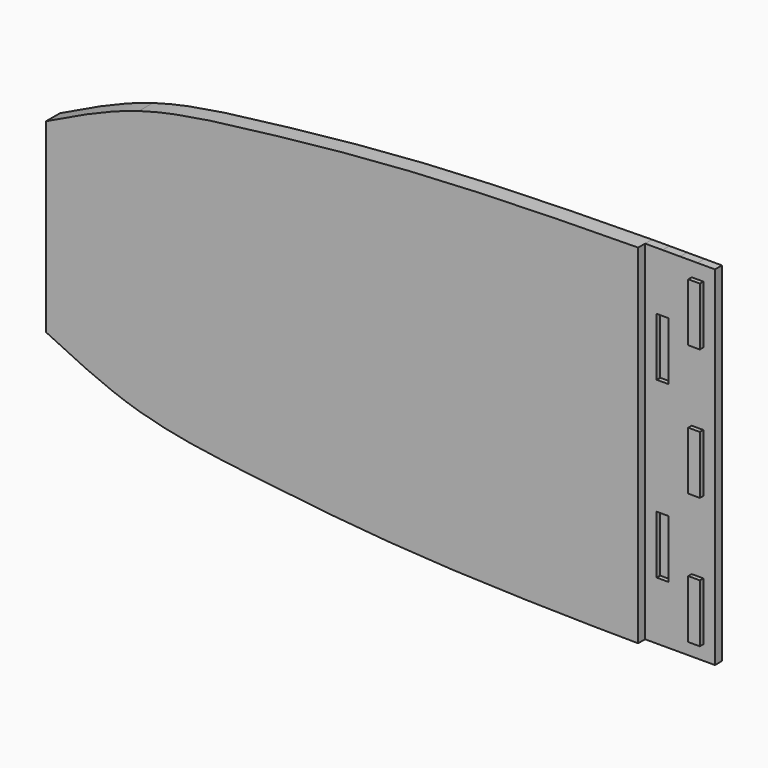
from build123d import *

# Parameters (mm, degrees)
F1_DEPTH = 19.05
F2_DEPTH = 9.525
F0_W     = 6.35
F0_H     = 63.5
F3_DEPTH = 4.7625
F0_H_2   = 31.75
F4_DEPTH = 14.2875


with BuildPart() as f1:
    # F0 (on Front) → F1 (new body)
    with BuildSketch(Plane.XZ):
        with BuildLine():
            Line((-722.3111987114, 1.2279e-06), (-620.7111987114, 1.2279e-06))
            Line((-620.7111987114, 1.2279e-06), (-620.7111987114, 144.4625012279))
            add(Edge.make_bspline(
                [(-722.3111987114, 101.6000012279), (-689.4180363188, 117.6879881372), (-656.5248739262, 133.7759750465), (-620.7111987114, 144.4625012279)],
                knots=[0, 0, 0, 0, 0.1537268507, 0.1537268507, 0.1537268507, 0.1537268507], degree=3))
            Line((-722.3111987114, 101.6000012279), (-722.3111987114, 1.2279e-06))
        make_face()
        with BuildLine():
            Line((-620.7111987114, 1.2279e-06), (-493.7111987114, 1.2279e-06))
            Line((-493.7111987114, 1.2279e-06), (-493.7111987114, 166.6875012279))
            add(Edge.make_bspline(
                [(-620.7111987114, 144.4625012279), (-581.9859047534, 156.0178321253), (-539.8459247327, 161.2577335799), (-493.7111987114, 166.6875012279)],
                knots=[0.1537268507, 0.1537268507, 0.1537268507, 0.1537268507, 0.3199515525, 0.3199515525, 0.3199515525, 0.3199515525], degree=3))
            Line((-620.7111987114, 144.4625012279), (-620.7111987114, 1.2279e-06))
        make_face()
        with BuildLine():
            Line((-620.7111987114, -144.4624987721), (-620.7111987114, 1.2279e-06))
            Line((-620.7111987114, 1.2279e-06), (-722.3111987114, 1.2279e-06))
            Line((-722.3111987114, 1.2279e-06), (-722.3111987114, -101.5999987721))
            add(Edge.make_bspline(
                [(-722.3111987114, -101.5999987721), (-689.4182841733, -117.6941564691), (-656.5253696352, -133.7883141661), (-620.7111987114, -144.4624987721)],
                knots=[0, 0, 0, 0, 0.1537255771, 0.1537255771, 0.1537255771, 0.1537255771], degree=3))
        make_face()
        with BuildLine():
            Line((-493.7111987114, -166.6874987721), (-493.7111987114, 1.2279e-06))
            Line((-493.7111987114, 1.2279e-06), (-620.7111987114, 1.2279e-06))
            Line((-620.7111987114, 1.2279e-06), (-620.7111987114, -144.4624987721))
            add(Edge.make_bspline(
                [(-620.7111987114, -144.4624987721), (-581.9853687438, -156.0044847356), (-539.8439833334, -161.2093964589), (-493.7111987114, -166.6874987721)],
                knots=[0.1537255771, 0.1537255771, 0.1537255771, 0.1537255771, 0.3199489018, 0.3199489018, 0.3199489018, 0.3199489018], degree=3))
        make_face()
        with BuildLine():
            Line((-290.9272084468, -185.0685181572), (-290.9272084468, -0.1247681572))
            Line((-290.9272084468, -0.1247681572), (-290.9272084468, 1.2279e-06))
            Line((-290.9272084468, 1.2279e-06), (-493.7111987114, 1.2279e-06))
            Line((-493.7111987114, 1.2279e-06), (-493.7111987114, -166.6874987721))
            add(Edge.make_bspline(
                [(-493.7111987114, -166.6874987721), (-435.736581071, -173.5717761816), (-371.4584655156, -180.8874953545), (-290.9272084468, -185.0685181572)],
                knots=[0.3199489018, 0.3199489018, 0.3199489018, 0.3199489018, 0.5288401224, 0.5288401224, 0.5288401224, 0.5288401224], degree=3))
        make_face()
        with BuildLine():
            Line((-493.7111987114, 1.2279e-06), (-290.9272084468, 1.2279e-06))
            Line((-290.9272084468, 1.2279e-06), (-290.9272084468, 184.8189818428))
            add(Edge.make_bspline(
                [(-493.7111987114, 166.6875012279), (-435.7373269286, 173.5106620133), (-371.4553650094, 180.633639874), (-290.9272084468, 184.8189818428)],
                knots=[0.3199515525, 0.3199515525, 0.3199515525, 0.3199515525, 0.528833026, 0.528833026, 0.528833026, 0.528833026], degree=3))
            Line((-493.7111987114, 166.6875012279), (-493.7111987114, 1.2279e-06))
        make_face()
        with BuildLine():
            Line((-290.9272084468, 184.8189818428), (-290.9272084468, 1.2279e-06))
            Line((-290.9272084468, 1.2279e-06), (-74.8163211554, 1.2279e-06))
            Line((-74.8163211554, 1.2279e-06), (-74.8163211554, 190.5000012279))
            add(Edge.make_bspline(
                [(-290.9272084468, 184.8189818428), (-207.9460116468, 189.1318172586), (-107.7137651743, 190.3253189595), (-74.8163211554, 190.5000012279)],
                knots=[0.528833026, 0.528833026, 0.528833026, 0.528833026, 0.744077425, 0.744077425, 0.744077425, 0.744077425], degree=3))
        make_face()
        with BuildLine():
            Line((-290.9272084468, 1.2279e-06), (-290.9272084468, -0.1247681572))
            Line((-290.9272084468, -0.1247681572), (-290.9272084468, -185.0685181572))
            add(Edge.make_bspline(
                [(-290.9272084468, -185.0685181572), (-207.9486072246, -189.376602204), (-107.7139882364, -190.35656804), (-74.8163211554, -190.4999987721)],
                knots=[0.5288401224, 0.5288401224, 0.5288401224, 0.5288401224, 0.7440795453, 0.7440795453, 0.7440795453, 0.7440795453], degree=3))
            Line((-74.8163211554, -190.4999987721), (-74.8163211554, 1.2279e-06))
            Line((-74.8163211554, 1.2279e-06), (-290.9272084468, 1.2279e-06))
        make_face()
    extrude(amount=F1_DEPTH)

    # F0 (on Front) → F2 (join)
    with BuildSketch(Plane.XZ):
        Polygon((-74.8163211554, 190.5000012279), (-74.8163211554, 1.2279e-06), (-55.7663211554, 1.2279e-06), (-55.7663211554, 63.5000012279), (-62.1163211554, 63.5000012279), (-62.1163211554, 127.0000012279), (-55.7663211554, 127.0000012279), (-55.7663211554, 190.5000012279), align=None)
        with BuildLine():
            Line((-55.7663211554, 1.2279e-06), (-74.8163211554, 1.2279e-06))
            Line((-74.8163211554, 1.2279e-06), (-74.8163211554, -190.4999987721))
            add(Edge.make_bspline(
                [(-74.8163211554, -190.4999987721), (-65.0505687749, -190.5425765334), (-61.2186404836, -190.5114376797), (-55.7663211554, -190.4999987721)],
                knots=[0.7440795453, 0.7440795453, 0.7440795453, 0.7440795453, 0.8079738908, 0.8079738908, 0.8079738908, 0.8079738908], degree=3))
            Line((-55.7663211554, -190.4999987721), (-55.7663211554, -126.9999987721))
            Line((-55.7663211554, -126.9999987721), (-62.1163211554, -126.9999987721))
            Line((-62.1163211554, -126.9999987721), (-62.1163211554, -63.4999987721))
            Line((-62.1163211554, -63.4999987721), (-55.7663211554, -63.4999987721))
            Line((-55.7663211554, -63.4999987721), (-55.7663211554, 1.2279e-06))
        make_face()
        with BuildLine():
            Line((-55.7663211554, 63.5000012279), (-55.7663211554, 1.2279e-06))
            Line((-55.7663211554, 1.2279e-06), (-36.7163211554, 1.2279e-06))
            Line((-36.7163211554, 1.2279e-06), (-36.5111987114, 1.2279e-06))
            Line((-36.5111987114, 1.2279e-06), (-36.5111987114, 190.5000012279))
            add(Edge.make_bspline(
                [(-55.7663211554, 190.5000012279), (-50.284669262, 190.4859953489), (-43.1652773507, 190.4962397359), (-36.5111987114, 190.5000012279)],
                knots=[0.8079722998, 0.8079722998, 0.8079722998, 0.8079722998, 0.8722102503, 0.8722102503, 0.8722102503, 0.8722102503], degree=3))
            Line((-55.7663211554, 190.5000012279), (-55.7663211554, 127.0000012279))
            Line((-55.7663211554, 127.0000012279), (-49.4163211554, 127.0000012279))
            Line((-49.4163211554, 127.0000012279), (-49.4163211554, 63.5000012279))
            Line((-49.4163211554, 63.5000012279), (-55.7663211554, 63.5000012279))
        make_face()
        with BuildLine():
            Line((-36.7163211554, 1.2279e-06), (-55.7663211554, 1.2279e-06))
            Line((-55.7663211554, 1.2279e-06), (-55.7663211554, -63.4999987721))
            Line((-55.7663211554, -63.4999987721), (-49.4163211554, -63.4999987721))
            Line((-49.4163211554, -63.4999987721), (-49.4163211554, -126.9999987721))
            Line((-49.4163211554, -126.9999987721), (-55.7663211554, -126.9999987721))
            Line((-55.7663211554, -126.9999987721), (-55.7663211554, -190.4999987721))
            add(Edge.make_bspline(
                [(-55.7663211554, -190.4999987721), (-50.2847262742, -190.4884984448), (-43.1652926622, -190.4969101842), (-36.5111987114, -190.4999987721)],
                knots=[0.8079738908, 0.8079738908, 0.8079738908, 0.8079738908, 0.872211309, 0.872211309, 0.872211309, 0.872211309], degree=3))
            Line((-36.5111987114, -190.4999987721), (-36.5111987114, 1.2279e-06))
            Line((-36.5111987114, 1.2279e-06), (-36.7163211554, 1.2279e-06))
        make_face()
        with BuildLine():
            Line((-36.5111987114, 1.2279e-06), (-36.5111987114, -190.4999987721))
            add(Edge.make_bspline(
                [(-36.5111987114, -190.4999987721), (-29.8926422792, -190.5030708649), (-23.7344683022, -190.5008765129), (-17.4611987114, -190.4999987721)],
                knots=[0.872211309, 0.872211309, 0.872211309, 0.872211309, 0.9361056545, 0.9361056545, 0.9361056545, 0.9361056545], degree=3))
            Line((-17.4611987114, -190.4999987721), (-17.4611987114, -174.6249987721))
            Line((-17.4611987114, -174.6249987721), (-23.8111987114, -174.6249987721))
            Line((-23.8111987114, -174.6249987721), (-23.8111987114, -111.1249987721))
            Line((-23.8111987114, -111.1249987721), (-17.4611987114, -111.1249987721))
            Line((-17.4611987114, -111.1249987721), (-17.4611987114, -95.2499987721))
            Line((-17.4611987114, -95.2499987721), (-17.4611987114, -31.7499987721))
            Line((-17.4611987114, -31.7499987721), (-23.8111987114, -31.7499987721))
            Line((-23.8111987114, -31.7499987721), (-23.8111987114, 1.2279e-06))
            Line((-23.8111987114, 1.2279e-06), (-36.5111987114, 1.2279e-06))
        make_face()
        Polygon((-17.4611987114, 190.5000012279), (-36.5111987114, 190.5000012279), (-36.5111987114, 1.2279e-06), (-23.8111987114, 1.2279e-06), (-23.8111987114, 31.7500012279), (-17.4611987114, 31.7500012279), (-17.4611987114, 95.2500012279), (-17.4611987114, 111.1250012279), (-23.8111987114, 111.1250012279), (-23.8111987114, 174.6250012279), (-17.4611987114, 174.6250012279), align=None)
        with BuildLine():
            Line((-17.4611987114, -174.6249987721), (-17.4611987114, -190.4999987721))
            add(Edge.make_bspline(
                [(-17.4611987114, -190.4999987721), (-11.1879291206, -190.4991210314), (-4.799563916, -190.4995599018), (1.5888012886, -190.4999987721)],
                knots=[0.9361056545, 0.9361056545, 0.9361056545, 0.9361056545, 1, 1, 1, 1], degree=3))
            Line((1.5888012886, -190.4999987721), (1.5888012886, 1.2279e-06))
            Line((1.5888012886, 1.2279e-06), (-11.1111987114, 1.2279e-06))
            Line((-11.1111987114, 1.2279e-06), (-11.1111987114, -31.7499987721))
            Line((-11.1111987114, -31.7499987721), (-17.4611987114, -31.7499987721))
            Line((-17.4611987114, -31.7499987721), (-17.4611987114, -95.2499987721))
            Line((-17.4611987114, -95.2499987721), (-17.4611987114, -111.1249987721))
            Line((-17.4611987114, -111.1249987721), (-11.1111987114, -111.1249987721))
            Line((-11.1111987114, -111.1249987721), (-11.1111987114, -174.6249987721))
            Line((-11.1111987114, -174.6249987721), (-17.4611987114, -174.6249987721))
        make_face()
        with BuildLine():
            add(Edge.make_bspline(
                [(-17.4611987114, 190.5000012279), (-11.1879247692, 190.4989322556), (-4.7995617403, 190.4994667417), (1.5888012886, 190.5000012279)],
                knots=[0.9361051251, 0.9361051251, 0.9361051251, 0.9361051251, 1, 1, 1, 1], degree=3))
            Line((-17.4611987114, 190.5000012279), (-17.4611987114, 174.6250012279))
            Line((-17.4611987114, 174.6250012279), (-11.1111987114, 174.6250012279))
            Line((-11.1111987114, 174.6250012279), (-11.1111987114, 111.1250012279))
            Line((-11.1111987114, 111.1250012279), (-17.4611987114, 111.1250012279))
            Line((-17.4611987114, 111.1250012279), (-17.4611987114, 95.2500012279))
            Line((-17.4611987114, 95.2500012279), (-17.4611987114, 31.7500012279))
            Line((-17.4611987114, 31.7500012279), (-11.1111987114, 31.7500012279))
            Line((-11.1111987114, 31.7500012279), (-11.1111987114, 1.2279e-06))
            Line((-11.1111987114, 1.2279e-06), (1.5888012886, 1.2279e-06))
            Line((1.5888012886, 1.2279e-06), (1.5888012886, 190.5000012279))
        make_face()
        Polygon((-11.1111987114, 174.6250012279), (-17.4611987114, 174.6250012279), (-17.4611987114, 142.8750012279), (-17.4611987114, 111.1250012279), (-11.1111987114, 111.1250012279), align=None)
        Polygon((-17.4611987114, 142.8750012279), (-17.4611987114, 174.6250012279), (-23.8111987114, 174.6250012279), (-23.8111987114, 111.1250012279), (-17.4611987114, 111.1250012279), align=None)
    extrude(amount=F2_DEPTH)

    # F0 (on Front) → F3 (join)
    with BuildSketch(Plane.XZ):
        with Locations((-58.9413211554, -95.2499987721)):
            Rectangle(F0_W, F0_H)
        with Locations((-52.5913211554, -95.2499987721)):
            Rectangle(F0_W, F0_H)
        Polygon((-74.8163211554, 190.5000012279), (-74.8163211554, 1.2279e-06), (-55.7663211554, 1.2279e-06), (-55.7663211554, 63.5000012279), (-62.1163211554, 63.5000012279), (-62.1163211554, 127.0000012279), (-55.7663211554, 127.0000012279), (-55.7663211554, 190.5000012279), align=None)
        Polygon((-62.1163211554, 63.5000012279), (-55.7663211554, 63.5000012279), (-55.7663211554, 95.2500012279), (-55.7663211554, 127.0000012279), (-62.1163211554, 127.0000012279), align=None)
        with BuildLine():
            Line((-55.7663211554, 63.5000012279), (-55.7663211554, 1.2279e-06))
            Line((-55.7663211554, 1.2279e-06), (-36.7163211554, 1.2279e-06))
            Line((-36.7163211554, 1.2279e-06), (-36.5111987114, 1.2279e-06))
            Line((-36.5111987114, 1.2279e-06), (-36.5111987114, 190.5000012279))
            add(Edge.make_bspline(
                [(-55.7663211554, 190.5000012279), (-50.284669262, 190.4859953489), (-43.1652773507, 190.4962397359), (-36.5111987114, 190.5000012279)],
                knots=[0.8079722998, 0.8079722998, 0.8079722998, 0.8079722998, 0.8722102503, 0.8722102503, 0.8722102503, 0.8722102503], degree=3))
            Line((-55.7663211554, 190.5000012279), (-55.7663211554, 127.0000012279))
            Line((-55.7663211554, 127.0000012279), (-49.4163211554, 127.0000012279))
            Line((-49.4163211554, 127.0000012279), (-49.4163211554, 63.5000012279))
            Line((-49.4163211554, 63.5000012279), (-55.7663211554, 63.5000012279))
        make_face()
        Polygon((-55.7663211554, 95.2500012279), (-55.7663211554, 63.5000012279), (-49.4163211554, 63.5000012279), (-49.4163211554, 127.0000012279), (-55.7663211554, 127.0000012279), align=None)
    extrude(amount=F3_DEPTH)

    # F0 (on Front) → F4 (join)
    with BuildSketch(Plane.XZ):
        with Locations((-20.6361987114, 15.8750012279)):
            Rectangle(F0_W, F0_H_2)
        with Locations((-20.6361987114, -15.8749987721)):
            Rectangle(F0_W, F0_H_2)
        with Locations((-20.6361987114, -142.8749987721)):
            Rectangle(F0_W, F0_H)
        with Locations((-14.2861987114, -142.8749987721)):
            Rectangle(F0_W, F0_H)
        Polygon((-11.1111987114, 174.6250012279), (-17.4611987114, 174.6250012279), (-17.4611987114, 142.8750012279), (-17.4611987114, 111.1250012279), (-11.1111987114, 111.1250012279), align=None)
        Polygon((-17.4611987114, 142.8750012279), (-17.4611987114, 174.6250012279), (-23.8111987114, 174.6250012279), (-23.8111987114, 111.1250012279), (-17.4611987114, 111.1250012279), align=None)
        with Locations((-14.2861987114, 15.8750012279)):
            Rectangle(F0_W, F0_H_2)
        with Locations((-14.2861987114, -15.8749987721)):
            Rectangle(F0_W, F0_H_2)
    extrude(amount=F4_DEPTH)


solid = f1.part
